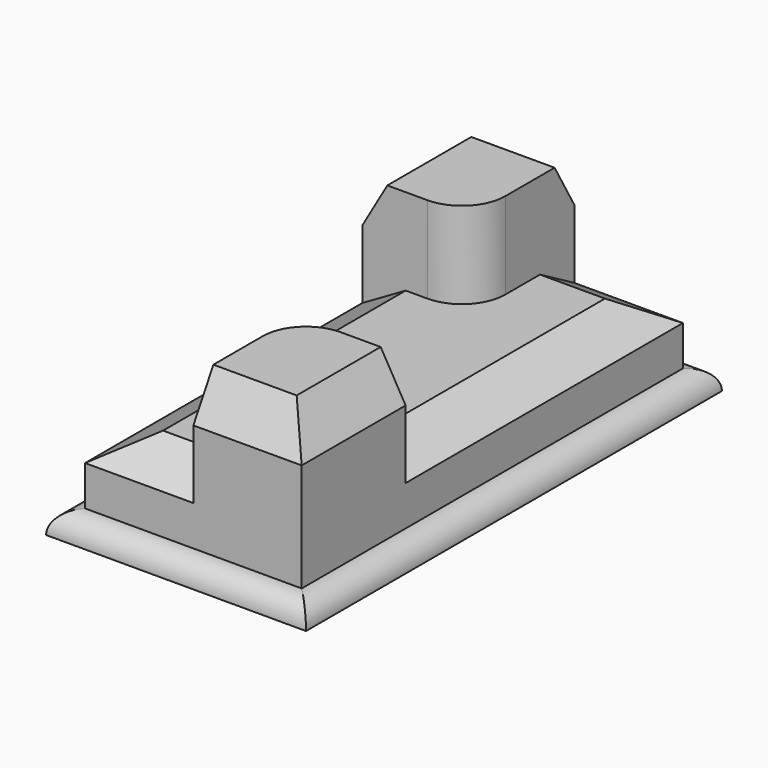
from build123d import *

# Parameters (mm, degrees)
F1_DEPTH    = 6.35
F2_DEPTH    = 25.4
F3_DEPTH    = 50.8
F4_C1_SIZE2 = 12.7
F4_C1_SIZE  = 7.3323484187
F4_C2_SIZE2 = 12.7
F4_C2_SIZE  = 7.3323484187
F5_SIZE2    = 7.3323484187
F5_SIZE     = 12.7
F6_SIZE2    = 7.3323484187
F6_SIZE     = 12.7
F7_R        = 6.34999


# Not quite as in the source:
# - a fillet or chamfer is up to 0.001 mm smaller than in the source, because OpenCascade refuses the exact size


with BuildPart() as f1:
    # F0 (on Top) → F1 (new body)
    with BuildSketch(Plane.XY):
        Polygon((44.45, 89.8741149127), (-31.75, 89.8741149127), (-31.75, 45.4241149127), (-31.75, -62.5258850873), (44.45, -62.5258850873), align=None)
        Polygon((-25.4, -56.1758850873), (-25.4, 45.4241149127), (-25.4, 83.5241149127), (6.35, 83.5241149127), (38.1, 83.5241149127), (38.1, -18.0758850873), (38.1, -56.1758850873), (6.35, -56.1758850873), align=None, mode=Mode.SUBTRACT)
    extrude(amount=F1_DEPTH)

    # F0 (on Top) → F2 (join)
    with BuildSketch(Plane.XY):
        with BuildLine():
            Line((-6.35, 45.4241149127), (-25.4, 45.4241149127))
            Line((-25.4, 45.4241149127), (-25.4, -56.1758850873))
            Line((-25.4, -56.1758850873), (6.35, -56.1758850873))
            Line((6.35, -56.1758850873), (6.35, -30.7758850873))
            ThreePointArc((6.35, -30.7758850873), (10.0697438789, -21.7956289662), (19.05, -18.0758850873))
            Line((19.05, -18.0758850873), (38.1, -18.0758850873))
            Line((38.1, -18.0758850873), (38.1, 83.5241149127))
            Line((38.1, 83.5241149127), (6.35, 83.5241149127))
            Line((6.35, 83.5241149127), (6.35, 58.1241149127))
            ThreePointArc((6.35, 58.1241149127), (2.6302561211, 49.1438587917), (-6.35, 45.4241149127))
        make_face()
    extrude(amount=F2_DEPTH)

    # F0 (on Top) → F3 (join)
    with BuildSketch(Plane.XY):
        with BuildLine():
            Line((-25.4, 83.5241149127), (-25.4, 45.4241149127))
            Line((-25.4, 45.4241149127), (-6.35, 45.4241149127))
            ThreePointArc((-6.35, 45.4241149127), (2.6302561211, 49.1438587917), (6.35, 58.1241149127))
            Line((6.35, 58.1241149127), (6.35, 83.5241149127))
            Line((6.35, 83.5241149127), (-25.4, 83.5241149127))
        make_face()
        with BuildLine():
            Line((6.35, -30.7758850873), (6.35, -56.1758850873))
            Line((6.35, -56.1758850873), (38.1, -56.1758850873))
            Line((38.1, -56.1758850873), (38.1, -18.0758850873))
            Line((38.1, -18.0758850873), (19.05, -18.0758850873))
            ThreePointArc((19.05, -18.0758850873), (10.0697438789, -21.7956289662), (6.35, -30.7758850873))
        make_face()
    extrude(amount=F3_DEPTH)

    # F4: chamfer of 12.7 x 7.3323484187 on 2 edges, made by hand

    # F4_c1
    f4_c1_edges = [f1.edges().sort_by_distance(p)[0] for p in [
        (-9.525, 83.5241149127, 50.8),
    ]]
    f4_c1_side = f1.faces().sort_by_distance((-9.525, 83.3774679444, 50.8))[0]
    chamfer(f4_c1_edges, length=F4_C1_SIZE, length2=F4_C1_SIZE2, reference=f4_c1_side)

    # F4_c2
    f4_c2_edges = [f1.edges().sort_by_distance(p)[0] for p in [
        (-25.4, 60.8079407034, 50.8),
    ]]
    f4_c2_side = f1.faces().sort_by_distance((-25.2533530316, 60.8079407034, 50.8))[0]
    chamfer(f4_c2_edges, length=F4_C2_SIZE, length2=F4_C2_SIZE2, reference=f4_c2_side)

    # F5
    f5_edges = [f1.edges().sort_by_distance(p)[0] for p in [
        (38.1, -37.125885, 50.8),
        (22.225, -56.175885, 50.8),
    ]]
    chamfer(f5_edges, length=F5_SIZE, length2=F5_SIZE2)

    # F6
    f6_edges = [f1.edges().sort_by_distance(p)[0] for p in [
        (-25.4, -5.375885, 25.4),
        (-9.525, -56.175885, 25.4),
        (38.1, 32.724115, 25.4),
        (22.225, 83.524115, 25.4),
    ]]
    f6_side = f1.faces().sort_by_distance((6.35, 13.674115, 25.4))[0]
    chamfer(f6_edges, length=F6_SIZE, length2=F6_SIZE2, reference=f6_side)

    # F7 (radius 6.35 in the source; OpenCascade refuses exactly that, so slightly less here)
    f7_edges = [f1.edges().sort_by_distance(p)[0] for p in [
        (44.45, 13.674115, 6.35),
        (6.35, -62.525885, 6.35),
        (-31.75, 13.674115, 6.35),
        (6.35, 89.874115, 6.35),
    ]]
    fillet(f7_edges, radius=F7_R)


solid = f1.part
